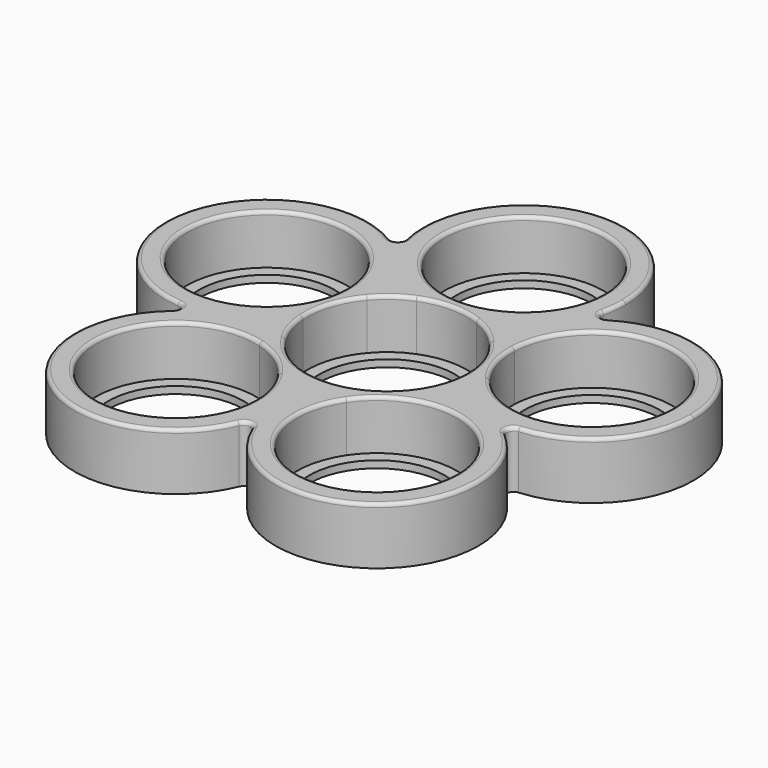
from build123d import *

# Parameters (mm, degrees)
F0_R     = 9.5
F1_DEPTH = 1
F2_DEPTH = 8
F3_R     = 1
F4_R     = 0.5


# Not quite as in the source:
# - a feature names something its author has since deleted; it is built from what else it names


with BuildPart() as f1:
    # F0 (on Top) → F1 (new body)
    with BuildSketch(Plane.XY):
        with BuildLine():
            ThreePointArc((10.2284120663, 14.0782014432), (9.495047993, 12.4528131318), (8.9704202214, 10.7485608828))
            ThreePointArc((8.9704202214, 10.7485608828), (10.4066054997, 9.3649646007), (11.6316340187, 7.7913471271))
            ThreePointArc((11.6316340187, 7.7913471271), (23.0128522969, 18.6148383481), (34.0253563911, 7.416407865))
            ThreePointArc((34.0253563911, 7.416407865), (26.4641809237, -3.175992997), (13.9898285303, 0.5335707014))
            ThreePointArc((13.9898285303, 0.5335707014), (13.9974569016, 0.266833821), (14, 0))
            ThreePointArc((14, 0), (13.8933608545, -1.7246808886), (13.5750679761, -3.4230877063))
            ThreePointArc((13.5750679761, -3.4230877063), (15.0012350971, -4.4934882713), (16.5499183742, -5.3773944508))
            ThreePointArc((16.5499183742, -5.3773944508), (18.5103382249, -5.8638525078), (20.3822840719, -6.6226055492))
            ThreePointArc((20.3822840719, -6.6226055492), (31.9972896511, -3.4894685452), (37.0753563911, 7.416407865))
            ThreePointArc((37.0753563911, 7.416407865), (28.1782821357, 20.6227959394), (12.5969443248, 17.3382064218))
            ThreePointArc((12.5969443248, 17.3382064218), (11.5284921698, 15.6240601548), (10.2284120663, 14.0782014432))
        make_face()
        with BuildLine():
            ThreePointArc((3.8156388718, 13.47), (5.6907926552, 12.7912031864), (7.4504765733, 11.8528645833))
            ThreePointArc((7.4504765733, 11.8528645833), (8.909197883, 12.8784581518), (10.2284120663, 14.0782014432))
            ThreePointArc((10.2284120663, 14.0782014432), (11.2968642212, 15.7923477102), (12.5969443248, 17.3382064218))
            ThreePointArc((12.5969443248, 17.3382064218), (13.8305631958, 20.5680877508), (14.25, 24))
            ThreePointArc((14.25, 24), (-3.4319122492, 37.8305631958), (-12.5969443248, 17.3382064218))
            ThreePointArc((-12.5969443248, 17.3382064218), (-11.2968642212, 15.7923477102), (-10.2284120663, 14.0782014432))
            ThreePointArc((-10.2284120663, 14.0782014432), (-8.909197883, 12.8784581518), (-7.4504765733, 11.8528645833))
            ThreePointArc((-7.4504765733, 11.8528645833), (-5.6907926552, 12.7912031864), (-3.8156388718, 13.47))
            ThreePointArc((-3.8156388718, 13.47), (-6.4305849126, 33.1699278995), (11.2, 24))
            ThreePointArc((11.2, 24), (9.1699278995, 17.5694150874), (3.8156388718, 13.47))
        make_face()
        with BuildLine():
            ThreePointArc((12.5969443248, 17.3382064218), (11.2968642212, 15.7923477102), (10.2284120663, 14.0782014432))
            ThreePointArc((10.2284120663, 14.0782014432), (11.5284921698, 15.6240601548), (12.5969443248, 17.3382064218))
        make_face()
        with BuildLine():
            ThreePointArc((16.5499183742, -5.3773944508), (14.7774602674, -5.1821963808), (12.9945011635, -5.2098886276))
            ThreePointArc((12.9945011635, -5.2098886276), (12.1224285616, -7.0033367597), (11.0043840401, -8.6546826573))
            ThreePointArc((11.0043840401, -8.6546826573), (20.840805716, -10.4668946222), (25.306846055, -19.416407865))
            ThreePointArc((25.306846055, -19.416407865), (10.8246599285, -30.1246875695), (4.8305506567, -13.1402351711))
            ThreePointArc((4.8305506567, -13.1402351711), (2.9145326225, -13.6932647529), (0.9393768355, -13.9684491323))
            ThreePointArc((0.9393768355, -13.9684491323), (0.3620752803, -15.6555866315), (0, -17.4016139847))
            ThreePointArc((0, -17.4016139847), (0.1073204046, -18.4064713036), (0.143153945, -19.416407865))
            ThreePointArc((0.143153945, -19.416407865), (0.1073204046, -20.4263444264), (0, -21.4312017453))
            ThreePointArc((0, -21.4312017453), (15.1167826164, -33.6305743246), (28.356846055, -19.416407865))
            ThreePointArc((28.356846055, -19.416407865), (26.1999740983, -11.8785862878), (20.3822840719, -6.6226055492))
            ThreePointArc((20.3822840719, -6.6226055492), (18.4218642212, -6.1361474922), (16.5499183742, -5.3773944508))
        make_face()
        with BuildLine():
            ThreePointArc((20.3822840719, -6.6226055492), (18.5103382249, -5.8638525078), (16.5499183742, -5.3773944508))
            ThreePointArc((16.5499183742, -5.3773944508), (18.4218642212, -6.1361474922), (20.3822840719, -6.6226055492))
        make_face()
        with BuildLine():
            ThreePointArc((-11.6316340187, 7.7913471271), (-10.4066054997, 9.3649646007), (-8.9704202214, 10.7485608828))
            ThreePointArc((-8.9704202214, 10.7485608828), (-9.495047993, 12.4528131318), (-10.2284120663, 14.0782014432))
            ThreePointArc((-10.2284120663, 14.0782014432), (-11.5284921698, 15.6240601548), (-12.5969443248, 17.3382064218))
            ThreePointArc((-12.5969443248, 17.3382064218), (-36.3779117483, 11.8199000348), (-20.3822840719, -6.6226055492))
            ThreePointArc((-20.3822840719, -6.6226055492), (-18.5103382249, -5.8638525078), (-16.5499183742, -5.3773944508))
            ThreePointArc((-16.5499183742, -5.3773944508), (-15.0012350971, -4.4934882713), (-13.5750679761, -3.4230877063))
            ThreePointArc((-13.5750679761, -3.4230877063), (-13.9237087836, -1.4595662745), (-13.9898285303, 0.5335707014))
            ThreePointArc((-13.9898285303, 0.5335707014), (-33.4771893736, 10.877398202), (-11.6316340187, 7.7913471271))
        make_face()
        with BuildLine():
            ThreePointArc((-12.5969443248, 17.3382064218), (-11.5284921698, 15.6240601548), (-10.2284120663, 14.0782014432))
            ThreePointArc((-10.2284120663, 14.0782014432), (-11.2968642212, 15.7923477102), (-12.5969443248, 17.3382064218))
        make_face()
        with BuildLine():
            ThreePointArc((0, -17.4016139847), (-0.3620752803, -15.6555866315), (-0.9393768355, -13.9684491323))
            ThreePointArc((-0.9393768355, -13.9684491323), (-2.9145326225, -13.6932647529), (-4.8305506567, -13.1402351711))
            ThreePointArc((-4.8305506567, -13.1402351711), (-3.3985663505, -16.1342217384), (-2.906846055, -19.416407865))
            ThreePointArc((-2.906846055, -19.416407865), (-23.0563592979, -26.150367526), (-11.0043840401, -8.6546826573))
            ThreePointArc((-11.0043840401, -8.6546826573), (-12.1224285616, -7.0033367597), (-12.9945011635, -5.2098886276))
            ThreePointArc((-12.9945011635, -5.2098886276), (-14.7774602674, -5.1821963808), (-16.5499183742, -5.3773944508))
            ThreePointArc((-16.5499183742, -5.3773944508), (-18.4218642212, -6.1361474922), (-20.3822840719, -6.6226055492))
            ThreePointArc((-20.3822840719, -6.6226055492), (-22.4827859002, -30.9449000348), (0, -21.4312017453))
            ThreePointArc((0, -21.4312017453), (-0.143153945, -19.416407865), (0, -17.4016139847))
        make_face()
        with BuildLine():
            ThreePointArc((0.143153945, -19.416407865), (0.1073204046, -18.4064713036), (0, -17.4016139847))
            ThreePointArc((0, -17.4016139847), (-0.143153945, -19.416407865), (0, -21.4312017453))
            ThreePointArc((0, -21.4312017453), (0.1073204046, -20.4263444264), (0.143153945, -19.416407865))
        make_face()
        with BuildLine():
            ThreePointArc((-20.3822840719, -6.6226055492), (-18.4218642212, -6.1361474922), (-16.5499183742, -5.3773944508))
            ThreePointArc((-16.5499183742, -5.3773944508), (-18.5103382249, -5.8638525078), (-20.3822840719, -6.6226055492))
        make_face()
        with BuildLine():
            ThreePointArc((11.1724197639, -0.7855167849), (9.2728010339, 3.0129156952), (8.5769622757, 7.202479998))
            ThreePointArc((8.5769622757, 7.202479998), (6.5831948257, 9.060990337), (4.1995384323, 10.3828645833))
            ThreePointArc((4.1995384323, 10.3828645833), (0, 9.75), (-4.1995384323, 10.3828645833))
            ThreePointArc((-4.1995384323, 10.3828645833), (-6.5831948257, 9.060990337), (-8.5769622757, 7.202479998))
            ThreePointArc((-8.5769622757, 7.202479998), (-9.2728010339, 3.0129156952), (-11.1724197639, -0.7855167849))
            ThreePointArc((-11.1724197639, -0.7855167849), (-10.6518329825, -3.460990337), (-9.5003926389, -5.9314871413))
            ThreePointArc((-9.5003926389, -5.9314871413), (-5.7309062099, -7.8879156952), (-2.7053967184, -10.8683406551))
            ThreePointArc((-2.7053967184, -10.8683406551), (0, -11.2), (2.7053967184, -10.8683406551))
            ThreePointArc((2.7053967184, -10.8683406551), (5.7309062099, -7.8879156952), (9.5003926389, -5.9314871413))
            ThreePointArc((9.5003926389, -5.9314871413), (10.6518329825, -3.460990337), (11.1724197639, -0.7855167849))
        make_face()
        Circle(F0_R, mode=Mode.SUBTRACT)
        with BuildLine():
            ThreePointArc((-3.8156388718, 13.47), (0, 12.8), (3.8156388718, 13.47))
            ThreePointArc((3.8156388718, 13.47), (0, 14), (-3.8156388718, 13.47))
        make_face()
        with BuildLine():
            ThreePointArc((-3.8156388718, 13.47), (0, 14), (3.8156388718, 13.47))
            ThreePointArc((3.8156388718, 13.47), (9.1699278995, 17.5694150874), (11.2, 24))
            ThreePointArc((11.2, 24), (-6.4305849126, 33.1699278995), (-3.8156388718, 13.47))
        make_face()
        with Locations((0, 24)):
            Circle(F0_R, mode=Mode.SUBTRACT)
        with BuildLine():
            ThreePointArc((-4.1995384323, 10.3828645833), (0, 11.2), (4.1995384323, 10.3828645833))
            ThreePointArc((4.1995384323, 10.3828645833), (5.8711955688, 11.015718634), (7.4504765733, 11.8528645833))
            ThreePointArc((7.4504765733, 11.8528645833), (5.6907926552, 12.7912031864), (3.8156388718, 13.47))
            ThreePointArc((3.8156388718, 13.47), (0, 12.8), (-3.8156388718, 13.47))
            ThreePointArc((-3.8156388718, 13.47), (-5.6907926552, 12.7912031864), (-7.4504765733, 11.8528645833))
            ThreePointArc((-7.4504765733, 11.8528645833), (-5.8711955688, 11.015718634), (-4.1995384323, 10.3828645833))
        make_face()
        with BuildLine():
            ThreePointArc((-4.1995384323, 10.3828645833), (0, 9.75), (4.1995384323, 10.3828645833))
            ThreePointArc((4.1995384323, 10.3828645833), (0, 11.2), (-4.1995384323, 10.3828645833))
        make_face()
        with BuildLine():
            ThreePointArc((-13.9898285303, 0.5335707014), (-13.3147912281, 4.3262379212), (-11.6316340187, 7.7913471271))
            ThreePointArc((-11.6316340187, 7.7913471271), (-33.4771893736, 10.877398202), (-13.9898285303, 0.5335707014))
        make_face()
        with Locations((-22.8253563911, 7.416407865)):
            Circle(F0_R, mode=Mode.SUBTRACT)
        with BuildLine():
            ThreePointArc((34.0253563911, 7.416407865), (23.0128522969, 18.6148383481), (11.6316340187, 7.7913471271))
            ThreePointArc((11.6316340187, 7.7913471271), (13.3147912281, 4.3262379212), (13.9898285303, 0.5335707014))
            ThreePointArc((13.9898285303, 0.5335707014), (26.4641809237, -3.175992997), (34.0253563911, 7.416407865))
        make_face()
        with Locations((22.8253563911, 7.416407865)):
            Circle(F0_R, mode=Mode.SUBTRACT)
        with BuildLine():
            ThreePointArc((25.306846055, -19.416407865), (20.840805716, -10.4668946222), (11.0043840401, -8.6546826573))
            ThreePointArc((11.0043840401, -8.6546826573), (8.2289935321, -11.3262379212), (4.8305506567, -13.1402351711))
            ThreePointArc((4.8305506567, -13.1402351711), (10.8246599285, -30.1246875695), (25.306846055, -19.416407865))
        make_face()
        with Locations((14.106846055, -19.416407865)):
            Circle(F0_R, mode=Mode.SUBTRACT)
        with BuildLine():
            ThreePointArc((-2.906846055, -19.416407865), (-3.3985663505, -16.1342217384), (-4.8305506567, -13.1402351711))
            ThreePointArc((-4.8305506567, -13.1402351711), (-8.2289935321, -11.3262379212), (-11.0043840401, -8.6546826573))
            ThreePointArc((-11.0043840401, -8.6546826573), (-23.0563592979, -26.150367526), (-2.906846055, -19.416407865))
        make_face()
        with Locations((-14.106846055, -19.416407865)):
            Circle(F0_R, mode=Mode.SUBTRACT)
        with BuildLine():
            ThreePointArc((-12.9945011635, -5.2098886276), (-13.3147912281, -4.3262379212), (-13.5750679761, -3.4230877063))
            ThreePointArc((-13.5750679761, -3.4230877063), (-15.0012350971, -4.4934882713), (-16.5499183742, -5.3773944508))
            ThreePointArc((-16.5499183742, -5.3773944508), (-14.7774602674, -5.1821963808), (-12.9945011635, -5.2098886276))
        make_face()
        with BuildLine():
            ThreePointArc((-9.5003926389, -5.9314871413), (-10.6518329825, -3.460990337), (-11.1724197639, -0.7855167849))
            ThreePointArc((-11.1724197639, -0.7855167849), (-12.2908701966, -2.179794541), (-13.5750679761, -3.4230877063))
            ThreePointArc((-13.5750679761, -3.4230877063), (-13.3147912281, -4.3262379212), (-12.9945011635, -5.2098886276))
            ThreePointArc((-12.9945011635, -5.2098886276), (-11.2247739489, -5.4609014114), (-9.5003926389, -5.9314871413))
        make_face()
        with BuildLine():
            ThreePointArc((-0.9393768355, -13.9684491323), (-1.724979964, -12.3629057488), (-2.7053967184, -10.8683406551))
            ThreePointArc((-2.7053967184, -10.8683406551), (-6.5831948257, -9.060990337), (-9.5003926389, -5.9314871413))
            ThreePointArc((-9.5003926389, -5.9314871413), (-11.2247739489, -5.4609014114), (-12.9945011635, -5.2098886276))
            ThreePointArc((-12.9945011635, -5.2098886276), (-12.1224285616, -7.0033367597), (-11.0043840401, -8.6546826573))
            ThreePointArc((-11.0043840401, -8.6546826573), (-7.5236512293, -10.355417528), (-4.8305506567, -13.1402351711))
            ThreePointArc((-4.8305506567, -13.1402351711), (-2.9145326225, -13.6932647529), (-0.9393768355, -13.9684491323))
        make_face()
        with BuildLine():
            ThreePointArc((-11.0043840401, -8.6546826573), (-8.2289935321, -11.3262379212), (-4.8305506567, -13.1402351711))
            ThreePointArc((-4.8305506567, -13.1402351711), (-7.5236512293, -10.355417528), (-11.0043840401, -8.6546826573))
        make_face()
        with BuildLine():
            ThreePointArc((-9.5003926389, -5.9314871413), (-6.5831948257, -9.060990337), (-2.7053967184, -10.8683406551))
            ThreePointArc((-2.7053967184, -10.8683406551), (-5.7309062099, -7.8879156952), (-9.5003926389, -5.9314871413))
        make_face()
        with BuildLine():
            ThreePointArc((-11.1724197639, -0.7855167849), (-10.6518329825, 3.460990337), (-8.5769622757, 7.202479998))
            ThreePointArc((-8.5769622757, 7.202479998), (-8.5757578679, 7.3094409178), (-8.5753563911, 7.416407865))
            ThreePointArc((-8.5753563911, 7.416407865), (-8.6744670124, 9.0941533138), (-8.9704202214, 10.7485608828))
            ThreePointArc((-8.9704202214, 10.7485608828), (-10.4066054997, 9.3649646007), (-11.6316340187, 7.7913471271))
            ThreePointArc((-11.6316340187, 7.7913471271), (-11.626925908, 7.6039037709), (-11.6253563911, 7.416407865))
            ThreePointArc((-11.6253563911, 7.416407865), (-12.2329555291, 3.7775833323), (-13.9898285303, 0.5335707014))
            ThreePointArc((-13.9898285303, 0.5335707014), (-13.9237087836, -1.4595662745), (-13.5750679761, -3.4230877063))
            ThreePointArc((-13.5750679761, -3.4230877063), (-12.2908701966, -2.179794541), (-11.1724197639, -0.7855167849))
        make_face()
        with BuildLine():
            ThreePointArc((-11.6253563911, 7.416407865), (-11.626925908, 7.6039037709), (-11.6316340187, 7.7913471271))
            ThreePointArc((-11.6316340187, 7.7913471271), (-13.3147912281, 4.3262379212), (-13.9898285303, 0.5335707014))
            ThreePointArc((-13.9898285303, 0.5335707014), (-12.2329555291, 3.7775833323), (-11.6253563911, 7.416407865))
        make_face()
        with BuildLine():
            ThreePointArc((-11.1724197639, -0.7855167849), (-9.2728010339, 3.0129156952), (-8.5769622757, 7.202479998))
            ThreePointArc((-8.5769622757, 7.202479998), (-10.6518329825, 3.460990337), (-11.1724197639, -0.7855167849))
        make_face()
        with BuildLine():
            ThreePointArc((-8.5769622757, 7.202479998), (-6.5831948257, 9.060990337), (-4.1995384323, 10.3828645833))
            ThreePointArc((-4.1995384323, 10.3828645833), (-5.8711955688, 11.015718634), (-7.4504765733, 11.8528645833))
            ThreePointArc((-7.4504765733, 11.8528645833), (-8.2289935321, 11.3262379212), (-8.9704202214, 10.7485608828))
            ThreePointArc((-8.9704202214, 10.7485608828), (-8.6744670124, 9.0941533138), (-8.5753563911, 7.416407865))
            ThreePointArc((-8.5753563911, 7.416407865), (-8.5757578679, 7.3094409178), (-8.5769622757, 7.202479998))
        make_face()
        with BuildLine():
            ThreePointArc((-8.9704202214, 10.7485608828), (-8.2289935321, 11.3262379212), (-7.4504765733, 11.8528645833))
            ThreePointArc((-7.4504765733, 11.8528645833), (-8.909197883, 12.8784581518), (-10.2284120663, 14.0782014432))
            ThreePointArc((-10.2284120663, 14.0782014432), (-9.495047993, 12.4528131318), (-8.9704202214, 10.7485608828))
        make_face()
        with BuildLine():
            ThreePointArc((4.1995384323, 10.3828645833), (6.5831948257, 9.060990337), (8.5769622757, 7.202479998))
            ThreePointArc((8.5769622757, 7.202479998), (8.6622717804, 8.9878830673), (8.9704202214, 10.7485608828))
            ThreePointArc((8.9704202214, 10.7485608828), (8.2289935321, 11.3262379212), (7.4504765733, 11.8528645833))
            ThreePointArc((7.4504765733, 11.8528645833), (5.8711955688, 11.015718634), (4.1995384323, 10.3828645833))
        make_face()
        with BuildLine():
            ThreePointArc((7.4504765733, 11.8528645833), (8.2289935321, 11.3262379212), (8.9704202214, 10.7485608828))
            ThreePointArc((8.9704202214, 10.7485608828), (9.495047993, 12.4528131318), (10.2284120663, 14.0782014432))
            ThreePointArc((10.2284120663, 14.0782014432), (8.909197883, 12.8784581518), (7.4504765733, 11.8528645833))
        make_face()
        with BuildLine():
            ThreePointArc((8.5769622757, 7.202479998), (10.5238295665, 3.8326245911), (11.2, 0))
            ThreePointArc((11.2, 0), (11.1931028173, -0.3930004099), (11.1724197639, -0.7855167849))
            ThreePointArc((11.1724197639, -0.7855167849), (12.2908701966, -2.179794541), (13.5750679761, -3.4230877063))
            ThreePointArc((13.5750679761, -3.4230877063), (13.8933608545, -1.7246808886), (14, 0))
            ThreePointArc((14, 0), (13.9974569016, 0.266833821), (13.9898285303, 0.5335707014))
            ThreePointArc((13.9898285303, 0.5335707014), (12.1735234086, 3.955417528), (11.6316340187, 7.7913471271))
            ThreePointArc((11.6316340187, 7.7913471271), (10.4066054997, 9.3649646007), (8.9704202214, 10.7485608828))
            ThreePointArc((8.9704202214, 10.7485608828), (8.6622717804, 8.9878830673), (8.5769622757, 7.202479998))
        make_face()
        with BuildLine():
            ThreePointArc((13.9898285303, 0.5335707014), (13.3147912281, 4.3262379212), (11.6316340187, 7.7913471271))
            ThreePointArc((11.6316340187, 7.7913471271), (12.1735234086, 3.955417528), (13.9898285303, 0.5335707014))
        make_face()
        with BuildLine():
            ThreePointArc((11.1724197639, -0.7855167849), (11.1931028173, -0.3930004099), (11.2, 0))
            ThreePointArc((11.2, 0), (10.5238295665, 3.8326245911), (8.5769622757, 7.202479998))
            ThreePointArc((8.5769622757, 7.202479998), (9.2728010339, 3.0129156952), (11.1724197639, -0.7855167849))
        make_face()
        with BuildLine():
            ThreePointArc((16.5499183742, -5.3773944508), (15.0012350971, -4.4934882713), (13.5750679761, -3.4230877063))
            ThreePointArc((13.5750679761, -3.4230877063), (13.3147912281, -4.3262379212), (12.9945011635, -5.2098886276))
            ThreePointArc((12.9945011635, -5.2098886276), (14.7774602674, -5.1821963808), (16.5499183742, -5.3773944508))
        make_face()
        with BuildLine():
            ThreePointArc((13.5750679761, -3.4230877063), (12.2908701966, -2.179794541), (11.1724197639, -0.7855167849))
            ThreePointArc((11.1724197639, -0.7855167849), (10.6518329825, -3.460990337), (9.5003926389, -5.9314871413))
            ThreePointArc((9.5003926389, -5.9314871413), (11.2247739489, -5.4609014114), (12.9945011635, -5.2098886276))
            ThreePointArc((12.9945011635, -5.2098886276), (13.3147912281, -4.3262379212), (13.5750679761, -3.4230877063))
        make_face()
        with BuildLine():
            ThreePointArc((12.9945011635, -5.2098886276), (11.2247739489, -5.4609014114), (9.5003926389, -5.9314871413))
            ThreePointArc((9.5003926389, -5.9314871413), (6.5831948257, -9.060990337), (2.7053967184, -10.8683406551))
            ThreePointArc((2.7053967184, -10.8683406551), (1.724979964, -12.3629057488), (0.9393768355, -13.9684491323))
            ThreePointArc((0.9393768355, -13.9684491323), (2.9145326225, -13.6932647529), (4.8305506567, -13.1402351711))
            ThreePointArc((4.8305506567, -13.1402351711), (7.5236512293, -10.355417528), (11.0043840401, -8.6546826573))
            ThreePointArc((11.0043840401, -8.6546826573), (12.1224285616, -7.0033367597), (12.9945011635, -5.2098886276))
        make_face()
        with BuildLine():
            ThreePointArc((2.7053967184, -10.8683406551), (6.5831948257, -9.060990337), (9.5003926389, -5.9314871413))
            ThreePointArc((9.5003926389, -5.9314871413), (5.7309062099, -7.8879156952), (2.7053967184, -10.8683406551))
        make_face()
        with BuildLine():
            ThreePointArc((4.8305506567, -13.1402351711), (8.2289935321, -11.3262379212), (11.0043840401, -8.6546826573))
            ThreePointArc((11.0043840401, -8.6546826573), (7.5236512293, -10.355417528), (4.8305506567, -13.1402351711))
        make_face()
        with BuildLine():
            ThreePointArc((0.9393768355, -13.9684491323), (1.724979964, -12.3629057488), (2.7053967184, -10.8683406551))
            ThreePointArc((2.7053967184, -10.8683406551), (0, -11.2), (-2.7053967184, -10.8683406551))
            ThreePointArc((-2.7053967184, -10.8683406551), (-1.724979964, -12.3629057488), (-0.9393768355, -13.9684491323))
            ThreePointArc((-0.9393768355, -13.9684491323), (0, -14), (0.9393768355, -13.9684491323))
        make_face()
        with BuildLine():
            ThreePointArc((0, -17.4016139847), (0.3620752803, -15.6555866315), (0.9393768355, -13.9684491323))
            ThreePointArc((0.9393768355, -13.9684491323), (0, -14), (-0.9393768355, -13.9684491323))
            ThreePointArc((-0.9393768355, -13.9684491323), (-0.3620752803, -15.6555866315), (0, -17.4016139847))
        make_face()
    extrude(amount=F1_DEPTH)

    # F0 (on Top) → F2 (join)
    with BuildSketch(Plane.XY):
        with BuildLine():
            ThreePointArc((7.4504765733, 11.8528645833), (8.2289935321, 11.3262379212), (8.9704202214, 10.7485608828))
            ThreePointArc((8.9704202214, 10.7485608828), (9.495047993, 12.4528131318), (10.2284120663, 14.0782014432))
            ThreePointArc((10.2284120663, 14.0782014432), (8.909197883, 12.8784581518), (7.4504765733, 11.8528645833))
        make_face()
        with BuildLine():
            ThreePointArc((10.2284120663, 14.0782014432), (9.495047993, 12.4528131318), (8.9704202214, 10.7485608828))
            ThreePointArc((8.9704202214, 10.7485608828), (10.4066054997, 9.3649646007), (11.6316340187, 7.7913471271))
            ThreePointArc((11.6316340187, 7.7913471271), (23.0128522969, 18.6148383481), (34.0253563911, 7.416407865))
            ThreePointArc((34.0253563911, 7.416407865), (26.4641809237, -3.175992997), (13.9898285303, 0.5335707014))
            ThreePointArc((13.9898285303, 0.5335707014), (13.9974569016, 0.266833821), (14, 0))
            ThreePointArc((14, 0), (13.8933608545, -1.7246808886), (13.5750679761, -3.4230877063))
            ThreePointArc((13.5750679761, -3.4230877063), (15.0012350971, -4.4934882713), (16.5499183742, -5.3773944508))
            ThreePointArc((16.5499183742, -5.3773944508), (18.5103382249, -5.8638525078), (20.3822840719, -6.6226055492))
            ThreePointArc((20.3822840719, -6.6226055492), (31.9972896511, -3.4894685452), (37.0753563911, 7.416407865))
            ThreePointArc((37.0753563911, 7.416407865), (28.1782821357, 20.6227959394), (12.5969443248, 17.3382064218))
            ThreePointArc((12.5969443248, 17.3382064218), (11.5284921698, 15.6240601548), (10.2284120663, 14.0782014432))
        make_face()
        with BuildLine():
            ThreePointArc((8.5769622757, 7.202479998), (10.5238295665, 3.8326245911), (11.2, 0))
            ThreePointArc((11.2, 0), (11.1931028173, -0.3930004099), (11.1724197639, -0.7855167849))
            ThreePointArc((11.1724197639, -0.7855167849), (12.2908701966, -2.179794541), (13.5750679761, -3.4230877063))
            ThreePointArc((13.5750679761, -3.4230877063), (13.8933608545, -1.7246808886), (14, 0))
            ThreePointArc((14, 0), (13.9974569016, 0.266833821), (13.9898285303, 0.5335707014))
            ThreePointArc((13.9898285303, 0.5335707014), (12.1735234086, 3.955417528), (11.6316340187, 7.7913471271))
            ThreePointArc((11.6316340187, 7.7913471271), (10.4066054997, 9.3649646007), (8.9704202214, 10.7485608828))
            ThreePointArc((8.9704202214, 10.7485608828), (8.6622717804, 8.9878830673), (8.5769622757, 7.202479998))
        make_face()
        with BuildLine():
            ThreePointArc((4.1995384323, 10.3828645833), (6.5831948257, 9.060990337), (8.5769622757, 7.202479998))
            ThreePointArc((8.5769622757, 7.202479998), (8.6622717804, 8.9878830673), (8.9704202214, 10.7485608828))
            ThreePointArc((8.9704202214, 10.7485608828), (8.2289935321, 11.3262379212), (7.4504765733, 11.8528645833))
            ThreePointArc((7.4504765733, 11.8528645833), (5.8711955688, 11.015718634), (4.1995384323, 10.3828645833))
        make_face()
        with BuildLine():
            ThreePointArc((-4.1995384323, 10.3828645833), (0, 11.2), (4.1995384323, 10.3828645833))
            ThreePointArc((4.1995384323, 10.3828645833), (5.8711955688, 11.015718634), (7.4504765733, 11.8528645833))
            ThreePointArc((7.4504765733, 11.8528645833), (5.6907926552, 12.7912031864), (3.8156388718, 13.47))
            ThreePointArc((3.8156388718, 13.47), (0, 12.8), (-3.8156388718, 13.47))
            ThreePointArc((-3.8156388718, 13.47), (-5.6907926552, 12.7912031864), (-7.4504765733, 11.8528645833))
            ThreePointArc((-7.4504765733, 11.8528645833), (-5.8711955688, 11.015718634), (-4.1995384323, 10.3828645833))
        make_face()
        with BuildLine():
            ThreePointArc((3.8156388718, 13.47), (5.6907926552, 12.7912031864), (7.4504765733, 11.8528645833))
            ThreePointArc((7.4504765733, 11.8528645833), (8.909197883, 12.8784581518), (10.2284120663, 14.0782014432))
            ThreePointArc((10.2284120663, 14.0782014432), (11.2968642212, 15.7923477102), (12.5969443248, 17.3382064218))
            ThreePointArc((12.5969443248, 17.3382064218), (13.8305631958, 20.5680877508), (14.25, 24))
            ThreePointArc((14.25, 24), (-3.4319122492, 37.8305631958), (-12.5969443248, 17.3382064218))
            ThreePointArc((-12.5969443248, 17.3382064218), (-11.2968642212, 15.7923477102), (-10.2284120663, 14.0782014432))
            ThreePointArc((-10.2284120663, 14.0782014432), (-8.909197883, 12.8784581518), (-7.4504765733, 11.8528645833))
            ThreePointArc((-7.4504765733, 11.8528645833), (-5.6907926552, 12.7912031864), (-3.8156388718, 13.47))
            ThreePointArc((-3.8156388718, 13.47), (-6.4305849126, 33.1699278995), (11.2, 24))
            ThreePointArc((11.2, 24), (9.1699278995, 17.5694150874), (3.8156388718, 13.47))
        make_face()
        with BuildLine():
            ThreePointArc((-11.6316340187, 7.7913471271), (-10.4066054997, 9.3649646007), (-8.9704202214, 10.7485608828))
            ThreePointArc((-8.9704202214, 10.7485608828), (-9.495047993, 12.4528131318), (-10.2284120663, 14.0782014432))
            ThreePointArc((-10.2284120663, 14.0782014432), (-11.5284921698, 15.6240601548), (-12.5969443248, 17.3382064218))
            ThreePointArc((-12.5969443248, 17.3382064218), (-36.3779117483, 11.8199000348), (-20.3822840719, -6.6226055492))
            ThreePointArc((-20.3822840719, -6.6226055492), (-18.5103382249, -5.8638525078), (-16.5499183742, -5.3773944508))
            ThreePointArc((-16.5499183742, -5.3773944508), (-15.0012350971, -4.4934882713), (-13.5750679761, -3.4230877063))
            ThreePointArc((-13.5750679761, -3.4230877063), (-13.9237087836, -1.4595662745), (-13.9898285303, 0.5335707014))
            ThreePointArc((-13.9898285303, 0.5335707014), (-33.4771893736, 10.877398202), (-11.6316340187, 7.7913471271))
        make_face()
        with BuildLine():
            ThreePointArc((-8.5769622757, 7.202479998), (-6.5831948257, 9.060990337), (-4.1995384323, 10.3828645833))
            ThreePointArc((-4.1995384323, 10.3828645833), (-5.8711955688, 11.015718634), (-7.4504765733, 11.8528645833))
            ThreePointArc((-7.4504765733, 11.8528645833), (-8.2289935321, 11.3262379212), (-8.9704202214, 10.7485608828))
            ThreePointArc((-8.9704202214, 10.7485608828), (-8.6744670124, 9.0941533138), (-8.5753563911, 7.416407865))
            ThreePointArc((-8.5753563911, 7.416407865), (-8.5757578679, 7.3094409178), (-8.5769622757, 7.202479998))
        make_face()
        with BuildLine():
            ThreePointArc((-11.1724197639, -0.7855167849), (-10.6518329825, 3.460990337), (-8.5769622757, 7.202479998))
            ThreePointArc((-8.5769622757, 7.202479998), (-8.5757578679, 7.3094409178), (-8.5753563911, 7.416407865))
            ThreePointArc((-8.5753563911, 7.416407865), (-8.6744670124, 9.0941533138), (-8.9704202214, 10.7485608828))
            ThreePointArc((-8.9704202214, 10.7485608828), (-10.4066054997, 9.3649646007), (-11.6316340187, 7.7913471271))
            ThreePointArc((-11.6316340187, 7.7913471271), (-11.626925908, 7.6039037709), (-11.6253563911, 7.416407865))
            ThreePointArc((-11.6253563911, 7.416407865), (-12.2329555291, 3.7775833323), (-13.9898285303, 0.5335707014))
            ThreePointArc((-13.9898285303, 0.5335707014), (-13.9237087836, -1.4595662745), (-13.5750679761, -3.4230877063))
            ThreePointArc((-13.5750679761, -3.4230877063), (-12.2908701966, -2.179794541), (-11.1724197639, -0.7855167849))
        make_face()
        with BuildLine():
            ThreePointArc((-9.5003926389, -5.9314871413), (-10.6518329825, -3.460990337), (-11.1724197639, -0.7855167849))
            ThreePointArc((-11.1724197639, -0.7855167849), (-12.2908701966, -2.179794541), (-13.5750679761, -3.4230877063))
            ThreePointArc((-13.5750679761, -3.4230877063), (-13.3147912281, -4.3262379212), (-12.9945011635, -5.2098886276))
            ThreePointArc((-12.9945011635, -5.2098886276), (-11.2247739489, -5.4609014114), (-9.5003926389, -5.9314871413))
        make_face()
        with BuildLine():
            ThreePointArc((-0.9393768355, -13.9684491323), (-1.724979964, -12.3629057488), (-2.7053967184, -10.8683406551))
            ThreePointArc((-2.7053967184, -10.8683406551), (-6.5831948257, -9.060990337), (-9.5003926389, -5.9314871413))
            ThreePointArc((-9.5003926389, -5.9314871413), (-11.2247739489, -5.4609014114), (-12.9945011635, -5.2098886276))
            ThreePointArc((-12.9945011635, -5.2098886276), (-12.1224285616, -7.0033367597), (-11.0043840401, -8.6546826573))
            ThreePointArc((-11.0043840401, -8.6546826573), (-7.5236512293, -10.355417528), (-4.8305506567, -13.1402351711))
            ThreePointArc((-4.8305506567, -13.1402351711), (-2.9145326225, -13.6932647529), (-0.9393768355, -13.9684491323))
        make_face()
        with BuildLine():
            ThreePointArc((0, -17.4016139847), (-0.3620752803, -15.6555866315), (-0.9393768355, -13.9684491323))
            ThreePointArc((-0.9393768355, -13.9684491323), (-2.9145326225, -13.6932647529), (-4.8305506567, -13.1402351711))
            ThreePointArc((-4.8305506567, -13.1402351711), (-3.3985663505, -16.1342217384), (-2.906846055, -19.416407865))
            ThreePointArc((-2.906846055, -19.416407865), (-23.0563592979, -26.150367526), (-11.0043840401, -8.6546826573))
            ThreePointArc((-11.0043840401, -8.6546826573), (-12.1224285616, -7.0033367597), (-12.9945011635, -5.2098886276))
            ThreePointArc((-12.9945011635, -5.2098886276), (-14.7774602674, -5.1821963808), (-16.5499183742, -5.3773944508))
            ThreePointArc((-16.5499183742, -5.3773944508), (-18.4218642212, -6.1361474922), (-20.3822840719, -6.6226055492))
            ThreePointArc((-20.3822840719, -6.6226055492), (-22.4827859002, -30.9449000348), (0, -21.4312017453))
            ThreePointArc((0, -21.4312017453), (-0.143153945, -19.416407865), (0, -17.4016139847))
        make_face()
        with BuildLine():
            ThreePointArc((16.5499183742, -5.3773944508), (14.7774602674, -5.1821963808), (12.9945011635, -5.2098886276))
            ThreePointArc((12.9945011635, -5.2098886276), (12.1224285616, -7.0033367597), (11.0043840401, -8.6546826573))
            ThreePointArc((11.0043840401, -8.6546826573), (20.840805716, -10.4668946222), (25.306846055, -19.416407865))
            ThreePointArc((25.306846055, -19.416407865), (10.8246599285, -30.1246875695), (4.8305506567, -13.1402351711))
            ThreePointArc((4.8305506567, -13.1402351711), (2.9145326225, -13.6932647529), (0.9393768355, -13.9684491323))
            ThreePointArc((0.9393768355, -13.9684491323), (0.3620752803, -15.6555866315), (0, -17.4016139847))
            ThreePointArc((0, -17.4016139847), (0.1073204046, -18.4064713036), (0.143153945, -19.416407865))
            ThreePointArc((0.143153945, -19.416407865), (0.1073204046, -20.4263444264), (0, -21.4312017453))
            ThreePointArc((0, -21.4312017453), (15.1167826164, -33.6305743246), (28.356846055, -19.416407865))
            ThreePointArc((28.356846055, -19.416407865), (26.1999740983, -11.8785862878), (20.3822840719, -6.6226055492))
            ThreePointArc((20.3822840719, -6.6226055492), (18.4218642212, -6.1361474922), (16.5499183742, -5.3773944508))
        make_face()
        with BuildLine():
            ThreePointArc((0, -17.4016139847), (0.3620752803, -15.6555866315), (0.9393768355, -13.9684491323))
            ThreePointArc((0.9393768355, -13.9684491323), (0, -14), (-0.9393768355, -13.9684491323))
            ThreePointArc((-0.9393768355, -13.9684491323), (-0.3620752803, -15.6555866315), (0, -17.4016139847))
        make_face()
        with BuildLine():
            ThreePointArc((0.9393768355, -13.9684491323), (1.724979964, -12.3629057488), (2.7053967184, -10.8683406551))
            ThreePointArc((2.7053967184, -10.8683406551), (0, -11.2), (-2.7053967184, -10.8683406551))
            ThreePointArc((-2.7053967184, -10.8683406551), (-1.724979964, -12.3629057488), (-0.9393768355, -13.9684491323))
            ThreePointArc((-0.9393768355, -13.9684491323), (0, -14), (0.9393768355, -13.9684491323))
        make_face()
        with BuildLine():
            ThreePointArc((-12.9945011635, -5.2098886276), (-13.3147912281, -4.3262379212), (-13.5750679761, -3.4230877063))
            ThreePointArc((-13.5750679761, -3.4230877063), (-15.0012350971, -4.4934882713), (-16.5499183742, -5.3773944508))
            ThreePointArc((-16.5499183742, -5.3773944508), (-14.7774602674, -5.1821963808), (-12.9945011635, -5.2098886276))
        make_face()
        with BuildLine():
            ThreePointArc((-8.9704202214, 10.7485608828), (-8.2289935321, 11.3262379212), (-7.4504765733, 11.8528645833))
            ThreePointArc((-7.4504765733, 11.8528645833), (-8.909197883, 12.8784581518), (-10.2284120663, 14.0782014432))
            ThreePointArc((-10.2284120663, 14.0782014432), (-9.495047993, 12.4528131318), (-8.9704202214, 10.7485608828))
        make_face()
        with BuildLine():
            ThreePointArc((16.5499183742, -5.3773944508), (15.0012350971, -4.4934882713), (13.5750679761, -3.4230877063))
            ThreePointArc((13.5750679761, -3.4230877063), (13.3147912281, -4.3262379212), (12.9945011635, -5.2098886276))
            ThreePointArc((12.9945011635, -5.2098886276), (14.7774602674, -5.1821963808), (16.5499183742, -5.3773944508))
        make_face()
        with BuildLine():
            ThreePointArc((13.5750679761, -3.4230877063), (12.2908701966, -2.179794541), (11.1724197639, -0.7855167849))
            ThreePointArc((11.1724197639, -0.7855167849), (10.6518329825, -3.460990337), (9.5003926389, -5.9314871413))
            ThreePointArc((9.5003926389, -5.9314871413), (11.2247739489, -5.4609014114), (12.9945011635, -5.2098886276))
            ThreePointArc((12.9945011635, -5.2098886276), (13.3147912281, -4.3262379212), (13.5750679761, -3.4230877063))
        make_face()
        with BuildLine():
            ThreePointArc((12.9945011635, -5.2098886276), (11.2247739489, -5.4609014114), (9.5003926389, -5.9314871413))
            ThreePointArc((9.5003926389, -5.9314871413), (6.5831948257, -9.060990337), (2.7053967184, -10.8683406551))
            ThreePointArc((2.7053967184, -10.8683406551), (1.724979964, -12.3629057488), (0.9393768355, -13.9684491323))
            ThreePointArc((0.9393768355, -13.9684491323), (2.9145326225, -13.6932647529), (4.8305506567, -13.1402351711))
            ThreePointArc((4.8305506567, -13.1402351711), (7.5236512293, -10.355417528), (11.0043840401, -8.6546826573))
            ThreePointArc((11.0043840401, -8.6546826573), (12.1224285616, -7.0033367597), (12.9945011635, -5.2098886276))
        make_face()
        with BuildLine():
            ThreePointArc((0.143153945, -19.416407865), (0.1073204046, -18.4064713036), (0, -17.4016139847))
            ThreePointArc((0, -17.4016139847), (-0.143153945, -19.416407865), (0, -21.4312017453))
            ThreePointArc((0, -21.4312017453), (0.1073204046, -20.4263444264), (0.143153945, -19.416407865))
        make_face()
        with BuildLine():
            ThreePointArc((-20.3822840719, -6.6226055492), (-18.4218642212, -6.1361474922), (-16.5499183742, -5.3773944508))
            ThreePointArc((-16.5499183742, -5.3773944508), (-18.5103382249, -5.8638525078), (-20.3822840719, -6.6226055492))
        make_face()
        with BuildLine():
            ThreePointArc((-12.5969443248, 17.3382064218), (-11.5284921698, 15.6240601548), (-10.2284120663, 14.0782014432))
            ThreePointArc((-10.2284120663, 14.0782014432), (-11.2968642212, 15.7923477102), (-12.5969443248, 17.3382064218))
        make_face()
        with BuildLine():
            ThreePointArc((12.5969443248, 17.3382064218), (11.2968642212, 15.7923477102), (10.2284120663, 14.0782014432))
            ThreePointArc((10.2284120663, 14.0782014432), (11.5284921698, 15.6240601548), (12.5969443248, 17.3382064218))
        make_face()
        with BuildLine():
            ThreePointArc((20.3822840719, -6.6226055492), (18.5103382249, -5.8638525078), (16.5499183742, -5.3773944508))
            ThreePointArc((16.5499183742, -5.3773944508), (18.4218642212, -6.1361474922), (20.3822840719, -6.6226055492))
        make_face()
    extrude(amount=F2_DEPTH)

    # F3
    f3_edges = [f1.edges().sort_by_distance(p)[0] for p in [
        (-20.382284, -6.622606, 4),
        (-12.596944, 17.338206, 4),
        (12.596944, 17.338206, 4),
        (20.382284, -6.622606, 4),
        (0, -21.431202, 4),
    ]]
    fillet(f3_edges, radius=F3_R)

    # F4
    f4_edges = [f1.edges().sort_by_distance(p)[0] for p in [
        (36.377912, 11.8199, 8),
        (-9.500393, 5.931487, 8),
        (31.660884, 14.299245, 8),
        (23.383141, -25.692581, 8),
        (3.815639, 34.53, 8),
        (-31.660884, 14.299245, 8),
        (-23.383141, -25.692581, 8),
    ]]
    fillet(f4_edges, radius=F4_R)


solid = f1.part
